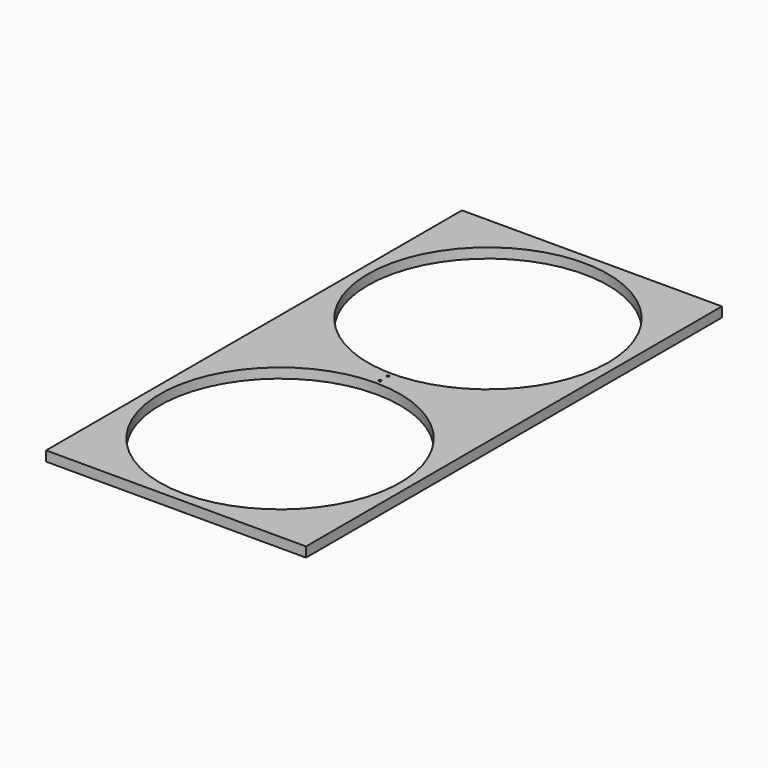
from build123d import *

# Parameters (mm, degrees)
F0_R     = 1.5875
F1_DEPTH = 12.7


with BuildPart() as f1:
    # F0 (on Top) → F1 (new body)
    with BuildSketch(Plane.XY):
        with BuildLine():
            ThreePointArc((4.517e-07, -333.375), (117.8658617487, -284.5533614293), (166.6875, -166.6875))
            Line((166.6875, -166.6875), (153.9875, -166.6875))
            ThreePointArc((153.9875, -166.6875), (0, -320.675), (-153.9875, -166.6875))
            Line((-153.9875, -166.6875), (-166.6875, -166.6875))
            ThreePointArc((-166.6875, -166.6875), (-117.8658614293, -284.5533617487), (4.517e-07, -333.375))
        make_face()
        with BuildLine():
            Line((153.9875, 166.6875), (166.6875, 166.6875))
            ThreePointArc((166.6875, 166.6875), (117.8658618859, 284.5533612921), (8.398e-07, 333.375))
            ThreePointArc((8.398e-07, 333.375), (-117.8658612921, 284.5533618859), (-166.6875, 166.6875))
            Line((-166.6875, 166.6875), (-153.9875, 166.6875))
            ThreePointArc((-153.9875, 166.6875), (0, 320.675), (153.9875, 166.6875))
        make_face()
        with BuildLine():
            ThreePointArc((-166.6875, -166.6875), (-117.865861589, -48.821638411), (0, 0))
            ThreePointArc((0, 0), (-117.865861589, 48.821638411), (-166.6875, 166.6875))
            Line((-166.6875, 166.6875), (-166.6875, -166.6875))
        make_face()
        with BuildLine():
            Line((153.9875, -166.6875), (166.6875, -166.6875))
            ThreePointArc((166.6875, -166.6875), (117.865861589, -48.821638411), (0, 0))
            Line((0, 0), (0, -4.7625))
            ThreePointArc((0, -4.7625), (1.1225320151, -5.2274679849), (1.5875, -6.35))
            ThreePointArc((1.5875, -6.35), (1.1225320151, -7.4725320151), (0, -7.9375))
            Line((0, -7.9375), (0, -12.7))
            ThreePointArc((0, -12.7), (108.885605468, -57.801894532), (153.9875, -166.6875))
        make_face()
        with BuildLine():
            ThreePointArc((0, 0), (117.865861589, 48.821638411), (166.6875, 166.6875))
            Line((166.6875, 166.6875), (153.9875, 166.6875))
            ThreePointArc((153.9875, 166.6875), (0, 12.7), (-153.9875, 166.6875))
            Line((-153.9875, 166.6875), (-166.6875, 166.6875))
            ThreePointArc((-166.6875, 166.6875), (-117.865861589, 48.821638411), (0, 0))
        make_face()
        with Locations((0, 6.35)):
            Circle(F0_R, mode=Mode.SUBTRACT)
        with BuildLine():
            ThreePointArc((0, 0), (117.865861589, -48.821638411), (166.6875, -166.6875))
            Line((166.6875, -166.6875), (166.6875, 166.6875))
            ThreePointArc((166.6875, 166.6875), (117.865861589, 48.821638411), (0, 0))
        make_face()
        with BuildLine():
            Line((-166.6875, -333.375), (4.517e-07, -333.375))
            ThreePointArc((4.517e-07, -333.375), (-117.8658614293, -284.5533617487), (-166.6875, -166.6875))
            Line((-166.6875, -166.6875), (-166.6875, -333.375))
        make_face()
        with BuildLine():
            Line((166.6875, -333.375), (166.6875, -166.6875))
            ThreePointArc((166.6875, -166.6875), (117.8658617487, -284.5533614293), (4.517e-07, -333.375))
            Line((4.517e-07, -333.375), (166.6875, -333.375))
        make_face()
        with BuildLine():
            ThreePointArc((-166.6875, 166.6875), (-117.8658612921, 284.5533618859), (8.398e-07, 333.375))
            Line((8.398e-07, 333.375), (-166.6875, 333.375))
            Line((-166.6875, 333.375), (-166.6875, 166.6875))
        make_face()
        with BuildLine():
            ThreePointArc((8.398e-07, 333.375), (117.8658618859, 284.5533612921), (166.6875, 166.6875))
            Line((166.6875, 166.6875), (166.6875, 333.375))
            Line((166.6875, 333.375), (8.398e-07, 333.375))
        make_face()
        with BuildLine():
            Line((0, -4.7625), (0, 0))
            ThreePointArc((0, 0), (-117.865861589, -48.821638411), (-166.6875, -166.6875))
            Line((-166.6875, -166.6875), (-153.9875, -166.6875))
            ThreePointArc((-153.9875, -166.6875), (-108.885605468, -57.801894532), (0, -12.7))
            Line((0, -12.7), (0, -7.9375))
            ThreePointArc((0, -7.9375), (-1.5875, -6.35), (0, -4.7625))
        make_face()
    extrude(amount=F1_DEPTH)


solid = f1.part
